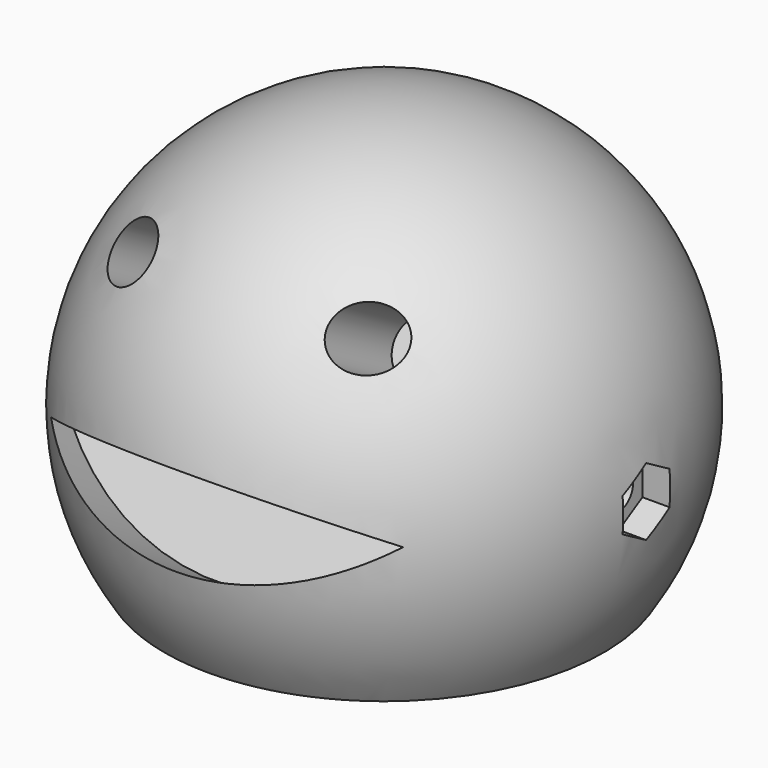
from build123d import *

# Parameters (mm, degrees)
F2_W      = 90.5019028811
F2_H      = 17.7580579312
F3_DEPTH  = 40
F5_DEPTH  = 20.25
F6_R      = 3
F7_DEPTH  = 50
F8_R      = 14
F11_R     = 5
F12_DEPTH = 40
F15_R     = 6
F16_DEPTH = 8
F18_DEPTH = 5


with BuildPart() as f1:
    # F0 (on Top) → F1 (revolve)
    with BuildSketch(Plane.XY):
        with BuildLine():
            Line((0, -45), (0, 45))
            ThreePointArc((0, 45), (-45, 0), (0, -45))
        make_face()
    revolve(axis=Axis((0, 2.1741483361, 0), (0, 1, 0)))

    # F2 (on Front) → F3 (cut, symmetric)
    with BuildSketch(Plane.XZ):
        with Locations((5.2887741476, -33.8790289656)):
            Rectangle(F2_W, F2_H)
    extrude(amount=F3_DEPTH, both=True, mode=Mode.SUBTRACT)

    # F4 (on Front) → F5 (cut, symmetric)
    with BuildSketch(Plane.XZ):
        with BuildLine():
            Line((-20.25, 5), (-20.25, -54.200690622))
            Line((-20.25, -54.200690622), (20.25, -54.200690622))
            Line((20.25, -54.200690622), (20.25, 5))
            ThreePointArc((20.25, 5), (0, -15.25), (-20.25, 5))
        make_face()
        with BuildLine():
            ThreePointArc((20.25, 5), (0, 25.25), (-20.25, 5))
            Line((-20.25, 5), (20.25, 5))
        make_face()
        with BuildLine():
            Line((20.25, 5), (-20.25, 5))
            ThreePointArc((-20.25, 5), (0, -15.25), (20.25, 5))
        make_face()
    extrude(amount=F5_DEPTH, both=True, mode=Mode.SUBTRACT)

    # F6 (on Right) → F7 (cut, symmetric)
    with BuildSketch(Plane.YZ):
        Circle(F6_R)
    extrude(amount=F7_DEPTH, both=True, mode=Mode.SUBTRACT)

    # F8
    f8_edges = [f1.edges().sort_by_distance(p)[0] for p in [
        (-20.25, -20.25, -10),
        (-20.25, 20.25, -10),
        (20.25, -20.25, -10),
        (20.25, 20.25, -10),
        (0, -20.25, 25.25),
        (0, 20.25, 25.25),
    ]]
    fillet(f8_edges, radius=F8_R)

    # F11 (on face) → F12 (cut)
    with BuildSketch(Plane(origin=(0, -56.3237066798, 32.5185072133), x_dir=(1, 0, 0), z_dir=(0, -0.8660254038, 0.5))):
        with BuildLine():
            Line((30, -15), (-30, -15))
            ThreePointArc((-30, -15), (0, -28.2363828336), (30, -15))
        make_face()
        with Locations((-20, 10)):
            Circle(F11_R)
        with Locations((20, 10)):
            Circle(F11_R)
    extrude(amount=-F12_DEPTH, mode=Mode.SUBTRACT)

    # F15 (on offset) → F16 (cut)
    with BuildSketch(Plane.YZ.offset(-45)):
        Circle(F15_R)
    extrude(amount=F16_DEPTH, mode=Mode.SUBTRACT)

    # F17 (on offset) → F18 (cut)
    with BuildSketch(Plane.YZ.offset(45)):
        Polygon((5, -2.8867513459), (5, 2.8867513459), (0, 5.7735026919), (-5, 2.8867513459), (-5, -2.8867513459), (0, -5.7735026919), align=None)
    extrude(amount=-F18_DEPTH, mode=Mode.SUBTRACT)


solid = f1.part
